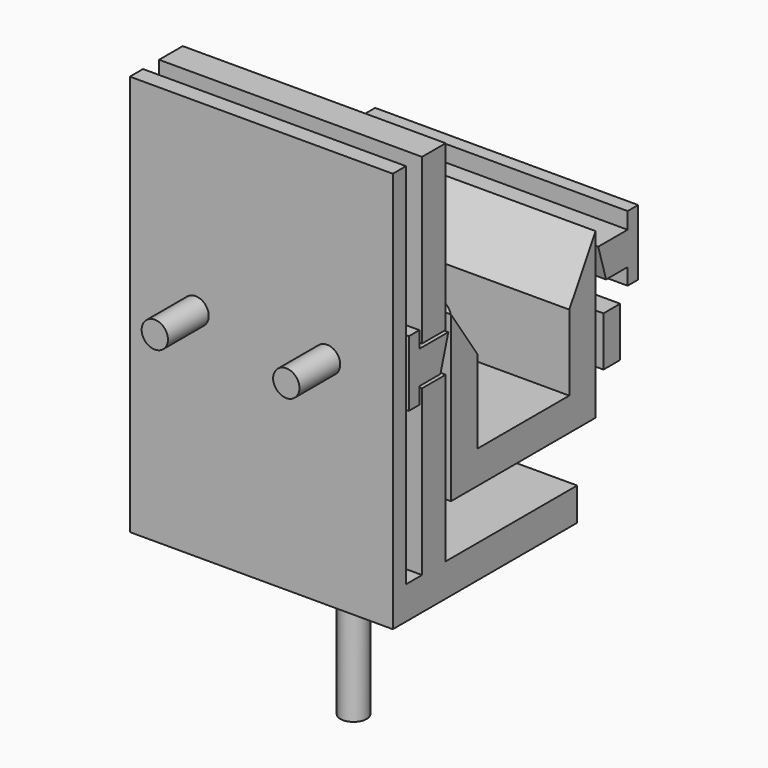
from build123d import *

# Parameters (mm, degrees)
F1_DEPTH = 80
F0_W     = 9
F0_H     = 50
F0_W_2   = 6.1117671594
F0_H_2   = 10
F0_W_3   = 6.3699182272
F0_H_3   = 15.0621980429
F2_R     = 4
F4_DEPTH = 36.3
F5_START = -111
F5_DEPTH = 89
F6_START = -80
F6_DEPTH = 22
F7_R     = 4
F8_DEPTH = 50
F7_R_2   = 10.5
F9_DEPTH = 10


# Not quite as in the source:
# - a feature of the source that left no trace in its solid (it failed there, or was rolled back) is left out


with BuildPart() as f1:
    # F0 (on Right) → F1 (new body)
    with BuildSketch(Plane.YZ):
        Polygon((115.7712601885, -159.0363204131), (160.7712601885, -159.0363204131), (160.7712601885, -149.0363204131), (125.7712601885, -149.0363204131), (115.7712601885, -149.0363204131), align=None)
        Polygon((115.7712601885, -149.0363204131), (125.7712601885, -149.0363204131), (125.7712601885, -123.6247909078), (115.7712601885, -109.0363204131), align=None)
        Polygon((170.7712601885, -159.0363204131), (170.7712601885, -109.0363204131), (160.7712601885, -125.9965002537), (160.7712601885, -149.0363204131), (160.7712601885, -159.0363204131), align=None)
    extrude(amount=F1_DEPTH)


with BuildPart() as f1b:
    # F0 (on Right) → F1, piece 2 (new body)
    with BuildSketch(Plane.YZ):
        with Locations((109.2712601885, -87.3286305666)):
            Rectangle(F0_W, F0_H)
    extrude(amount=F1_DEPTH)


with BuildPart() as f1c:
    # F0 (on Right) → F1, piece 3 (new body)
    with BuildSketch(Plane.YZ):
        Polygon((103.7712601885, -128.3286305666), (103.7712601885, -123.3286305666), (111.7712601885, -123.3286305666), (114.7712601885, -113.3286305666), (103.7712601885, -113.3286305666), (103.7712601885, -108.3286305666), (99.7712601885, -108.3286305666), (99.7712601885, -128.3286305666), align=None)
    extrude(amount=F1_DEPTH)

    # F2 (on face) → F6 (join)
    with BuildSketch(Plane(origin=(0, 180.1411784157, 0), x_dir=(-1, 0, 0), z_dir=(0, 1, 0)).offset(F6_START)):
        with Locations((-60, -118.6247909078)):
            Circle(F2_R)
        with Locations((-20, -118.6247909078)):
            Circle(F2_R)
    extrude(amount=-F6_DEPTH)


with BuildPart() as f1d:
    # F0 (on Right) → F1, piece 4 (new body)
    with BuildSketch(Plane.YZ):
        with Locations((109.2712601885, -149.3286305666)):
            Rectangle(F0_W, F0_H)
        Polygon((163.7621800169, -174.3286305666), (113.7712601885, -174.3286305666), (104.7712601885, -174.3286305666), (104.7712601885, -184.3286305666), (163.7621800169, -184.3286305666), align=None)
        Polygon((98.6594930291, -184.3286305666), (98.6594930291, -174.3286305666), (98.6594930291, -62.3286305666), (93.6594930291, -62.3286305666), (93.6594930291, -184.3286305666), align=None)
        with Locations((101.7153766088, -179.3286305666)):
            Rectangle(F0_W_2, F0_H_2)
    extrude(amount=F1_DEPTH)

    # F7 (on face) → F8 (join)
    with BuildSketch(Plane(origin=(0, 0, -184.3286305666), x_dir=(1, 0, 0), z_dir=(0, 0, -1))):
        with Locations((40, -128.710836523)):
            Circle(F7_R)
    extrude(amount=F8_DEPTH)

    # F7 (on face) → F9 (join)
    with BuildSketch(Plane(origin=(0, 0, -184.3286305666), x_dir=(1, 0, 0), z_dir=(0, 0, -1))):
        with Locations((40, -128.710836523)):
            Circle(F7_R_2)
        with Locations((40, -128.710836523)):
            Circle(F7_R, mode=Mode.SUBTRACT)
        with Locations((40, -128.710836523)):
            Circle(F7_R)
    extrude(amount=F9_DEPTH)


with BuildPart() as f1e:
    # F0 (on Right) → F1, piece 5 (new body)
    with BuildSketch(Plane.YZ):
        Polygon((186.9528900847, -128.6247909078), (186.9528900847, -108.6247909078), (182.9528900847, -108.6247909078), (182.9528900847, -113.6247909078), (171.7712601885, -113.6247909078), (174.7712601885, -123.6247909078), (182.9528900847, -123.6247909078), (182.9528900847, -128.6247909078), align=None)
    extrude(amount=F1_DEPTH)


with BuildPart() as f1f:
    # F0 (on Right) → F1, piece 6 (new body)
    with BuildSketch(Plane.YZ):
        with Locations((176.9562193021, -139.8249312887)):
            Rectangle(F0_W_3, F0_H_3)
    extrude(amount=F1_DEPTH)


with BuildPart() as f4_tool:
    # F2 (on face) → F4 (new body)
    with BuildSketch(Plane(origin=(0, 180.1411784157, 0), x_dir=(-1, 0, 0), z_dir=(0, 1, 0))):
        with Locations((-40, -139.8249312887)):
            Circle(F2_R)
    extrude(amount=-F4_DEPTH)


with BuildPart() as f1_1:
    add(f1.part)

    # F4: cut by f4_tool
    add(f4_tool.part, mode=Mode.SUBTRACT)

    # F2 (on face) → F5 (cut)
    with BuildSketch(Plane(origin=(0, 180.1411784157, 0), x_dir=(-1, 0, 0), z_dir=(0, 1, 0)).offset(F5_START)):
        with Locations((-60, -118.6247909078)):
            Circle(F2_R)
        with Locations((-20, -118.6247909078)):
            Circle(F2_R)
    extrude(amount=-F5_DEPTH, mode=Mode.SUBTRACT)


with BuildPart() as f1f_1:
    add(f1f.part)

    # F4: cut by f4_tool
    add(f4_tool.part, mode=Mode.SUBTRACT)


solid = Compound([f1b.part, f1c.part, f1d.part, f1e.part, f1_1.part, f1f_1.part])
